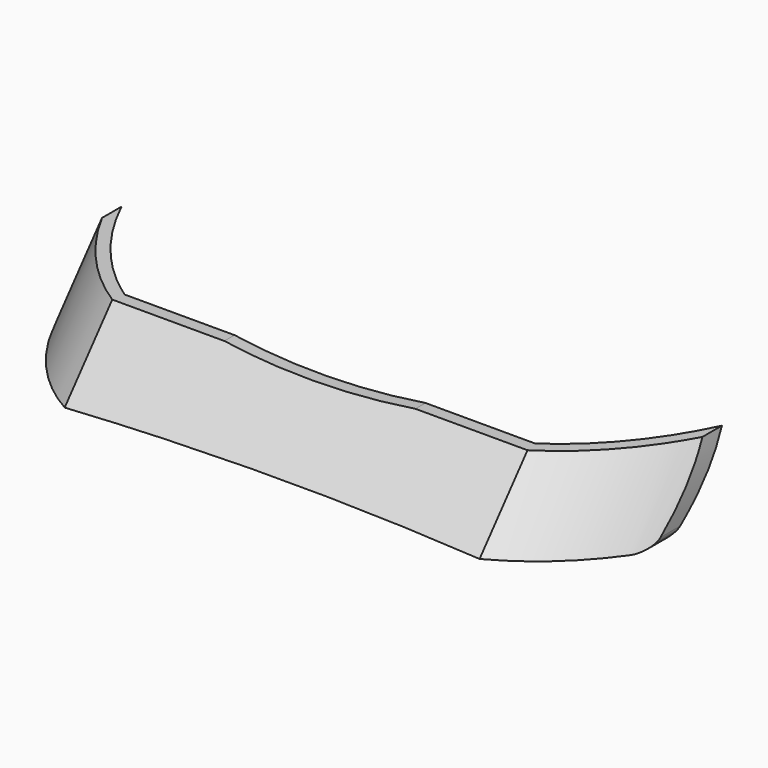
from build123d import *

# Parameters (mm, degrees)
F1_DEPTH      = 40
F1_DEPTH_BACK = 11
F4_DEPTH      = 35
F4_DEPTH_BACK = 27.9057510197
F5_T1_DEPTH   = 14.5743949702
F5_T3_DEPTH   = 14.6258479297


# Not quite as in the source:
# - a fillet or chamfer that OpenCascade refuses, or shapes differently, is made with other operations: its cross-section is extruded or revolved along the edge and cut away or added


with BuildPart() as f1:
    # F0 (on Front) → F1 (new body, two sides)
    with BuildSketch(Plane.XZ) as f1_sk:
        with BuildLine():
            Line((-19.5, 15.5), (-61.5, 15.5))
            ThreePointArc((-61.5, 15.5), (-62.0026261084, 7.75), (-61.5, 0))
            ThreePointArc((-61.5, 0), (-0.0044648026, 1.8801470046), (61.5, 0.319182139))
            ThreePointArc((61.5, 0.319182139), (62.0026261084, 8.069182139), (61.5, 15.819182139))
            Line((61.5, 15.819182139), (19.5, 15.819182139))
            ThreePointArc((19.5, 15.819182139), (0.0077989053, 14.7066639823), (-19.5, 15.5))
        make_face()
    extrude(amount=F1_DEPTH)
    extrude(f1_sk.sketch, amount=-F1_DEPTH_BACK)

    # F3 (on face) → F4 (cut, two sides)
    with BuildSketch(Plane(origin=(0, -8.7376098383, -10.4130779155), x_dir=(1, 0, 0), z_dir=(0, -0.6427876097, -0.7660444431))) as f4_sk:
        with BuildLine():
            Line((41.9965417924, 21), (0, 20.9813332936))
            Line((0, 20.9813332936), (-42.034011751, 20.9813332936))
            ThreePointArc((-42.034011751, 20.9813332936), (-55.2445439017, 11.0585633209), (-64.5, -2.6277822851))
            Line((-64.5, -2.6277822851), (-64.5, -10.626510717))
            Line((-64.5, -10.626510717), (-64.5, -28.2158330083))
            Line((-64.5, -28.2158330083), (0, -28.2158330083))
            Line((0, -28.2158330083), (64.5, -28.2158330083))
            Line((64.5, -28.2158330083), (64.5, -12.4673116952))
            Line((64.5, -12.4673116952), (64.5, -2.6264255467))
            ThreePointArc((64.5, -2.6264255467), (55.2297238243, 11.0740614176), (41.9965417924, 21))
        make_face()
        with BuildLine():
            Line((64.5, 1.9813332936), (64.5, 22.9813332936))
            Line((64.5, 22.9813332936), (64.5, 52.9813332936))
            Line((64.5, 52.9813332936), (-64.5, 52.9813332936))
            Line((-64.5, 52.9813332936), (-64.5, 22.9813332936))
            Line((-64.5, 22.9813332936), (-64.5, 1.9813332936))
            ThreePointArc((-64.5, 1.9813332936), (-55.1354627813, 14.1946752549), (-42.5, 22.9813332936))
            Line((-42.5, 22.9813332936), (42.5, 22.9813332936))
            ThreePointArc((42.5, 22.9813332936), (55.1354627813, 14.1946752549), (64.5, 1.9813332936))
        make_face()
    extrude(amount=-F4_DEPTH, mode=Mode.SUBTRACT)
    extrude(f4_sk.sketch, amount=F4_DEPTH_BACK, mode=Mode.SUBTRACT)

    # F5: fillet of radius 2 on 2 edges, made by hand

    # F5_s2 → F5_t1 (cut)
    with BuildSketch(Plane.XZ.offset(-1.1764499881)):
        with BuildLine():
            ThreePointArc((61.7168527659, 2.2201536136), (61.0312003552, 0.8993903708), (59.6231546265, 0.4177868017))
            ThreePointArc((59.6231546265, 0.4177868017), (60.5615983725, 0.3688853121), (61.5, 0.319182139))
            ThreePointArc((61.5, 0.319182139), (61.6160042169, 1.2688034371), (61.7168527659, 2.2201536136))
        make_face()
    extrude(amount=F5_T1_DEPTH, mode=Mode.SUBTRACT)

    # F5_s4 → F5_t3 (cut)
    with BuildSketch(Plane.XZ.offset(-0.9347638385)):
        with BuildLine():
            ThreePointArc((-59.6137615285, 0.1089088503), (-61.0283512081, 0.5866856233), (-61.7178391039, 1.9110500173))
            ThreePointArc((-61.7178391039, 1.9110500173), (-61.6165778825, 0.9546520415), (-61.5, 0))
            ThreePointArc((-61.5, 0), (-60.5569041472, 0.0548594049), (-59.6137615285, 0.1089088503))
        make_face()
    extrude(amount=F5_T3_DEPTH, mode=Mode.SUBTRACT)


solid = f1.part
